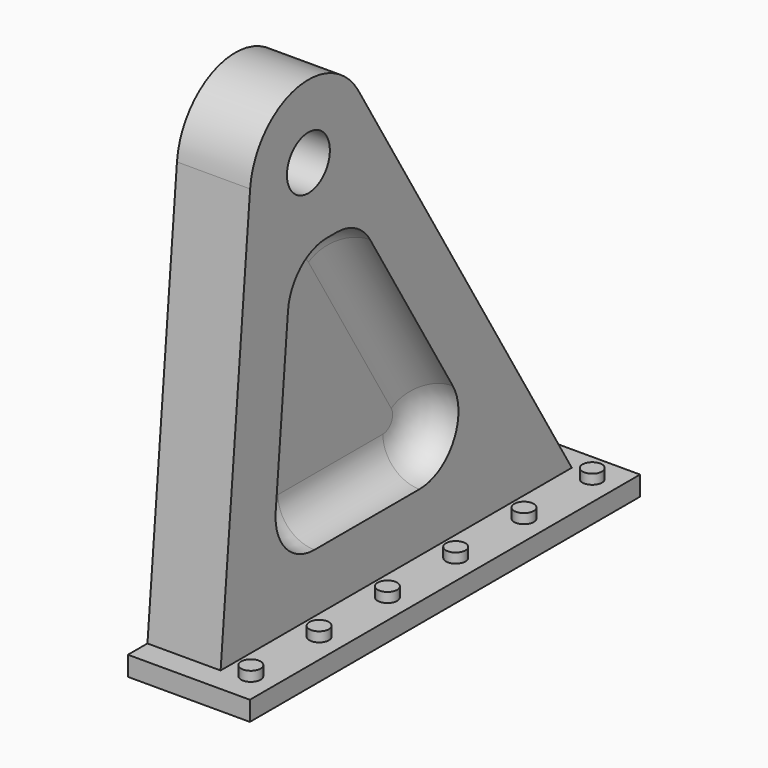
from build123d import *

# Parameters (mm, degrees)
F0_W     = 20
F0_H     = 0.8
F1_DEPTH = 5
F2_R     = 1.1
F3_DEPTH = 3
F5_DEPTH = 1.5
F6_R     = 2
F7_R     = 1.49999
F8_R     = 0.4
F9_DEPTH = 0.4


# Not quite as in the source:
# - a fillet or chamfer is up to 0.001 mm smaller than in the source, because OpenCascade refuses the exact size


with BuildPart() as f1:
    # F0 (on Right) → F1 (new body)
    with BuildSketch(Plane.YZ):
        with Locations((4.5, 0.4)):
            Rectangle(F0_W, F0_H)
    extrude(amount=F1_DEPTH)

    # F2 (on Right) → F3 (join)
    with BuildSketch(Plane.YZ):
        with BuildLine():
            Line((-4.5, 0.8), (13.5, 0.8))
            Line((13.5, 0.8), (2.5660948526, 18.8540776067))
            ThreePointArc((2.5660948526, 18.8540776067), (-0.6760626552, 20.2228306975), (-2.9878775484, 17.5694211496))
            Line((-2.9878775484, 17.5694211496), (-4.5, 0.8))
        make_face()
        with Locations((0, 17.3)):
            Circle(F2_R, mode=Mode.SUBTRACT)
    extrude(amount=F3_DEPTH)

    # F4 (on face) → F5 (cut)
    with BuildSketch(Plane.YZ.offset(3)):
        Polygon((-0.8819657168, 14.2), (-1.8738512935, 3.2), (9.2406928099, 3.2), (2.5788760591, 14.2), align=None)
    extrude(amount=-F5_DEPTH, mode=Mode.SUBTRACT)

    # F6
    f6_edges = [f1.edges().sort_by_distance(p)[0] for p in [
        (2.25, -0.881966, 14.2),
        (2.25, 2.578876, 14.2),
        (2.25, 9.240693, 3.2),
        (2.25, -1.873851, 3.2),
    ]]
    fillet(f6_edges, radius=F6_R)

    # F7 (radius 1.5 in the source; OpenCascade refuses exactly that, so slightly less here)
    f7_edges = [f1.edges().sort_by_distance(p)[0] for p in [
        (1.5, 5.282331, 9.736052),
        (1.5, 7.433697, 4.218191),
        (1.5, 2.433741, 13.942427),
        (1.5, 3.002938, 3.2),
        (1.5, 1.198869, 14.2),
        (1.5, -1.161746, 3.850783),
        (1.5, -0.403411, 13.676352),
        (1.5, -1.361712, 8.879614),
    ]]
    fillet(f7_edges, radius=F7_R)

    # F8 (on face) → F9 (join)
    with BuildSketch(Plane.XY.offset(0.8)):
        with Locations((4, 13.3)):
            Circle(F8_R)
        with Locations((4, 9.7999986556)):
            Circle(F8_R)
        with Locations((4, 6.2999973111)):
            Circle(F8_R)
        with Locations((4, 2.7999959667)):
            Circle(F8_R)
        with Locations((4, -0.7000053778)):
            Circle(F8_R)
        with Locations((4, -4.2000067222)):
            Circle(F8_R)
    extrude(amount=F9_DEPTH)


solid = f1.part
